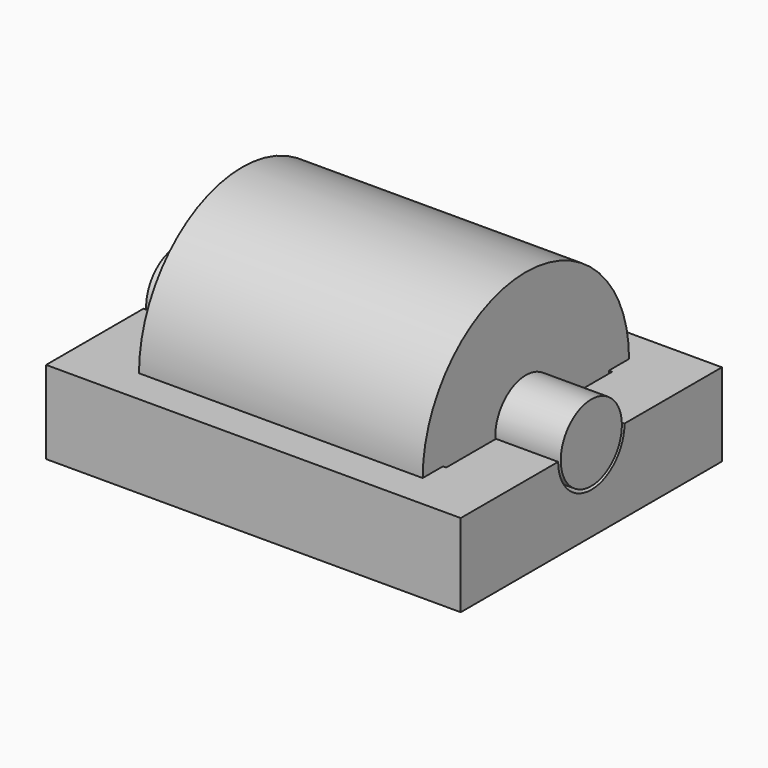
from build123d import *

# Parameters (mm, degrees)
F1_DEPTH      = 6.35
F1_DEPTH_BACK = 6.35
F2_W          = 8.89
F2_H          = 1.905
F2_H_2        = 2.54
F3_DEPTH      = 2.54
F4_R          = 1.17
F5_DEPTH      = 6.35
F5_DEPTH_BACK = 6.35
F6_R          = 3.95
F7_DEPTH      = 4.345
F7_DEPTH_BACK = 4.345


with BuildPart() as f1:
    # F0 (on Right) → F1 (new body, two sides)
    with BuildSketch(Plane.YZ) as f1_sk:
        with BuildLine():
            Line((-5, 0), (0, 0))
            Line((0, 0), (5, 0))
            Line((5, 0), (5, 2.54))
            Line((5, 2.54), (1.27, 2.54))
            ThreePointArc((1.27, 2.54), (0, 1.27), (-1.27, 2.54))
            Line((-1.27, 2.54), (-5, 2.54))
            Line((-5, 2.54), (-5, 0))
        make_face()
    extrude(amount=F1_DEPTH)
    extrude(f1_sk.sketch, amount=-F1_DEPTH_BACK)

    # F2 (on Top) → F3 (cut, through all)
    with BuildSketch(Plane.XY):
        with Locations((0, -2.2225)):
            Rectangle(F2_W, F2_H)
        Rectangle(F2_W, F2_H_2)
        with Locations((0, 2.2225)):
            Rectangle(F2_W, F2_H)
    extrude(amount=F3_DEPTH, mode=Mode.SUBTRACT)


with BuildPart() as f5:
    # F4 (on Right) → F5 (new body, two sides)
    with BuildSketch(Plane.YZ) as f5_sk:
        with Locations((0, 2.54)):
            Circle(F4_R)
    extrude(amount=F5_DEPTH)
    extrude(f5_sk.sketch, amount=-F5_DEPTH_BACK)

    # F6 (on Right) → F7 (join, two sides)
    with BuildSketch(Plane.YZ) as f7_sk:
        with Locations((0, 2.54)):
            Circle(F6_R)
    extrude(amount=F7_DEPTH)
    extrude(f7_sk.sketch, amount=-F7_DEPTH_BACK)


solid = Compound([f1.part, f5.part])
